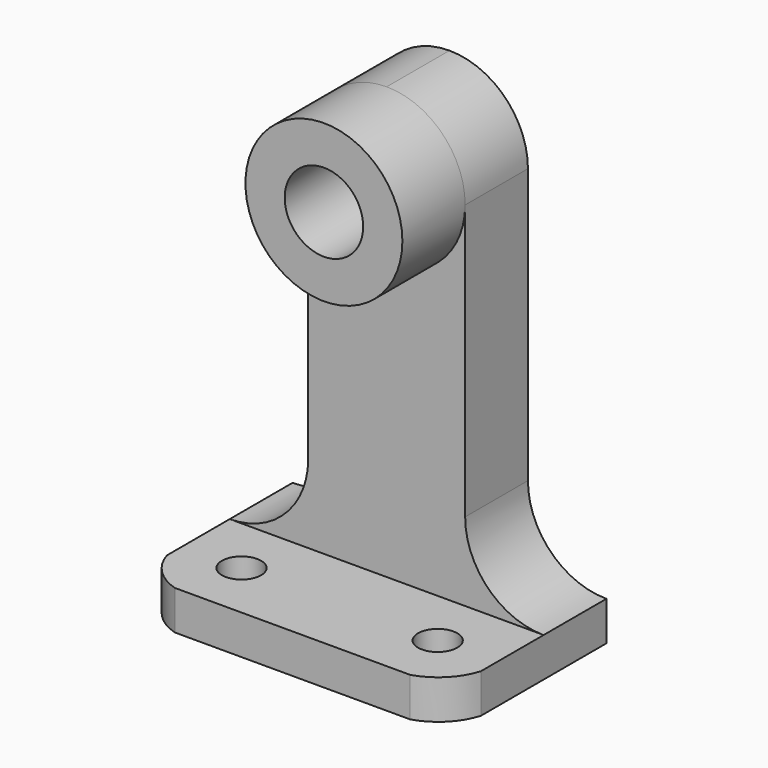
from build123d import *
from build123d import SkipClean  # not in build123d's __all__

# Parameters (mm, degrees)
F1_DEPTH  = 12.7
F2_W      = 50.8
F2_H      = 6.35
F3_DEPTH  = 19.05
F5_DEPTH  = 12.7
F7_R      = 12.7
F8_DEPTH  = 25.4
F9_R      = 6.35
F10_DEPTH = 25.4
F11_R     = 3.175
F12_DEPTH = 6.35


with BuildPart() as f1:
    # F0 (on Front) → F1 (new body)
    with BuildSketch(Plane.XZ):
        Polygon((0, 19.05), (0, 0), (50.8, 0), (50.8, 19.05), (38.1, 19.05), (38.1, 76.2), (12.7, 76.2), (12.7, 19.05), align=None)
    extrude(amount=F1_DEPTH)

    # F2 (on face) → F3 (join)
    with BuildSketch(Plane.XZ.offset(12.7)):
        with Locations((25.4, 3.175)):
            Rectangle(F2_W, F2_H)
    extrude(amount=F3_DEPTH)

    # F4 (on face) → F5 (cut)
    with BuildSketch(Plane.XZ.offset(12.7)):
        with BuildLine():
            Line((0, 19.05), (0, 6.35))
            ThreePointArc((0, 6.35), (8.9802561211, 10.0697438789), (12.7, 19.05))
            Line((12.7, 19.05), (0, 19.05))
        make_face()
        with BuildLine():
            Line((50.8, 19.05), (38.1, 19.05))
            ThreePointArc((38.1, 19.05), (41.8197438789, 10.0697438789), (50.8, 6.35))
            Line((50.8, 6.35), (50.8, 19.05))
        make_face()
    extrude(amount=-F5_DEPTH, mode=Mode.SUBTRACT)

    # F7 (on Front) → F8 (join)
    with BuildSketch(Plane.XZ):
        with Locations((25.4, 63.5)):
            Circle(F7_R)
    extrude(amount=F8_DEPTH)

    # F9 (on face) + F8_face1 (on face) → F10 (cut)
    with BuildSketch(Plane.XZ.offset(25.4)):
        with Locations((25.4, 63.5)):
            Circle(F9_R)
    with BuildSketch(Plane(origin=(35.2632271754, -12.7, 73.3632271754), x_dir=(1, 0, 0), z_dir=(0, -1, 0))):
        with BuildLine():
            Line((2.8367728246, -9.8632271754), (2.8367728246, 2.8367728246))
            Line((2.8367728246, 2.8367728246), (-9.8632271754, 2.8367728246))
            ThreePointArc((-9.8632271754, 2.8367728246), (-0.8829710543, -0.8829710543), (2.8367728246, -9.8632271754))
        make_face()
        with BuildLine():
            ThreePointArc((-22.5632271754, -9.8632271754), (-18.8434832965, -0.8829710543), (-9.8632271754, 2.8367728246))
            Line((-9.8632271754, 2.8367728246), (-22.5632271754, 2.8367728246))
            Line((-22.5632271754, 2.8367728246), (-22.5632271754, -9.8632271754))
        make_face()
    with SkipClean():  # cleaning this boolean's faces spoils the solid; the shape is the same uncleaned
        extrude(amount=-F10_DEPTH, mode=Mode.SUBTRACT)

    # F6 (on face) + F11 (on face) → F12 (cut)
    with BuildSketch(Plane.XY.offset(6.35)):
        with BuildLine():
            Line((0, -31.75), (6.35, -31.75))
            ThreePointArc((6.35, -31.75), (2.3796890107, -29.3703109893), (0, -25.4))
            Line((0, -25.4), (0, -31.75))
        make_face()
        with BuildLine():
            ThreePointArc((50.8, -25.4), (48.4203109893, -29.3703109893), (44.45, -31.75))
            Line((44.45, -31.75), (50.8, -31.75))
            Line((50.8, -31.75), (50.8, -25.4))
        make_face()
    with BuildSketch(Plane.XY.offset(6.35)):
        with Locations((9.525, -22.225)):
            Circle(F11_R)
        with Locations((41.275, -22.225)):
            Circle(F11_R)
    with SkipClean():  # cleaning this boolean's faces spoils the solid; the shape is the same uncleaned
        extrude(amount=-F12_DEPTH, mode=Mode.SUBTRACT)


solid = f1.part
